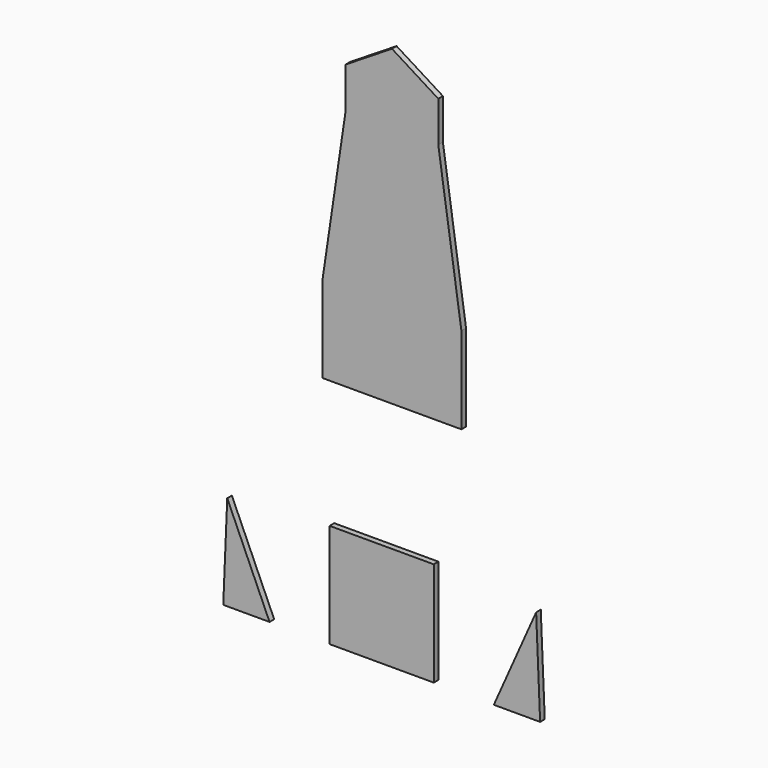
from build123d import *

# Parameters (mm, degrees)
F0_W     = 457.2
F0_H     = 457.2
F1_DEPTH = 25.4


# Not quite as in the source:
# - ends of sketch curves that miss each other by under 0.0002 mm in the source are joined


with BuildPart() as f1:
    # F0 (on Front) → F1 (new body)
    with BuildSketch(Plane.XZ):
        with Locations((-73.4027251601, 38.2703000127)):
            Rectangle(F0_W, F0_H)
    extrude(amount=F1_DEPTH)


with BuildPart() as f1b:
    # F0 (on Front) → F1, piece 2 (new body)
    with BuildSketch(Plane.XZ):
        Polygon((-768.841027844, -190.3296999873), (-565.641027844, -190.3296999873), (-751.3275345236, 227.4649400419), align=None)
    extrude(amount=F1_DEPTH)


with BuildPart() as f1c:
    # F0 (on Front) → F1, piece 3 (new body)
    with BuildSketch(Plane.XZ):
        Polygon((604.5220842033, 227.4649400419), (418.8355775237, -190.3296999873), (622.0355775237, -190.3296999873), align=None)
    extrude(amount=F1_DEPTH)


with BuildPart() as f1d:
    # F0 (on Front) → F1, piece 4 (new body)
    with BuildSketch(Plane.XZ):
        Polygon((-333.0557037953, 827.8134502805), (276.5442959808, 827.7969272853), (276.5442959808, 1208.7969272853), (174.944296007, 1894.604935298), (174.944296007, 2072.404935298), (-28.2561103925, 2199.4051892978), (-231.455703993, 2072.4009312714), (-231.455703993, 1894.6009312714), (-333.0557040787, 1208.7929232587), align=None)
    extrude(amount=F1_DEPTH)


solid = Compound([f1.part, f1b.part, f1c.part, f1d.part])
